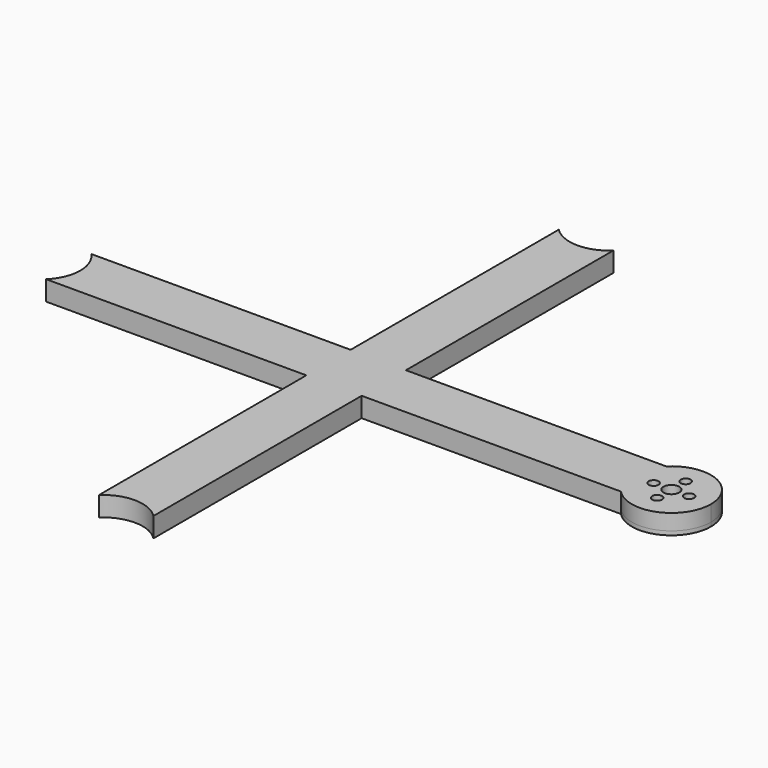
from build123d import *

# Parameters (mm, degrees)
F0_R     = 1.25
F0_R_2   = 2
F1_DEPTH = 5
F2_DEPTH = 1


with BuildPart() as f1:
    # F0 (on Top) → F1 (new body)
    with BuildSketch(Plane.XY):
        with BuildLine():
            ThreePointArc((72.7387571288, -6.8756346591), (83.7005115381, -9.2901137967), (90, 0))
            ThreePointArc((90, 0), (83.861757699, 9.2242521363), (72.9826345051, 7.1243653409))
            ThreePointArc((72.9826345051, 7.1243653409), (70.0015169041, 0.1741717018), (72.7387571288, -6.8756346591))
        make_face()
        with Locations((75.5, 0)):
            Circle(F0_R, mode=Mode.SUBTRACT)
        with Locations((80, -4.5)):
            Circle(F0_R, mode=Mode.SUBTRACT)
        with Locations((80, 0)):
            Circle(F0_R_2, mode=Mode.SUBTRACT)
        with Locations((84.5, 0)):
            Circle(F0_R, mode=Mode.SUBTRACT)
        with Locations((80, 4.5)):
            Circle(F0_R, mode=Mode.SUBTRACT)
        with BuildLine():
            ThreePointArc((72.7387571288, -6.8756346591), (70.0015169041, 0.1741717018), (72.9826345051, 7.1243653409))
            Line((72.9826345051, 7.1243653409), (7.1243653409, 7.1243653409))
            Line((7.1243653409, 7.1243653409), (7.1243653409, 0.2487306818))
            Line((7.1243653409, 0.2487306818), (7.1243653409, 0))
            Line((7.1243653409, 0), (7.1243653409, -6.8756346591))
            Line((7.1243653409, -6.8756346591), (72.7387571288, -6.8756346591))
        make_face()
        Polygon((7.1243653409, 0.2487306818), (7.1243653409, 7.1243653409), (0.2487306818, 7.1243653409), (0, 7.1243653409), (-6.8756346591, 7.1243653409), (-6.8756346591, 0.2487306818), (-6.8756346591, 0), (-6.8756346591, -6.8756346591), (0, -6.8756346591), (0.2487306818, -6.8756346591), (7.1243653409, -6.8756346591), (7.1243653409, 0), align=None)
        with BuildLine():
            Line((0.2487306818, 7.1243653409), (7.1243653409, 7.1243653409))
            Line((7.1243653409, 7.1243653409), (7.1243653409, 72.7387571288))
            ThreePointArc((7.1243653409, 72.7387571288), (0.0745589801, 70.0015169041), (-6.8756346591, 72.9826345051))
            Line((-6.8756346591, 72.9826345051), (-6.8756346591, 7.1243653409))
            Line((-6.8756346591, 7.1243653409), (0, 7.1243653409))
            Line((0, 7.1243653409), (0.2487306818, 7.1243653409))
        make_face()
        with BuildLine():
            Line((7.1243653409, -72.7339038233), (7.1243653409, -6.8756346591))
            Line((7.1243653409, -6.8756346591), (0.2487306818, -6.8756346591))
            Line((0.2487306818, -6.8756346591), (0, -6.8756346591))
            Line((0, -6.8756346591), (-6.8756346591, -6.8756346591))
            Line((-6.8756346591, -6.8756346591), (-6.8756346591, -72.4900264469))
            ThreePointArc((-6.8756346591, -72.4900264469), (0.1741717018, -69.7527862223), (7.1243653409, -72.7339038233))
        make_face()
        with BuildLine():
            Line((-6.8756346591, 0.2487306818), (-6.8756346591, 7.1243653409))
            Line((-6.8756346591, 7.1243653409), (-72.4900264469, 7.1243653409))
            ThreePointArc((-72.4900264469, 7.1243653409), (-70.4611555214, 3.94924222), (-69.7512693182, 0.2487306818))
            ThreePointArc((-69.7512693182, 0.2487306818), (-70.5270171818, -3.6130270171), (-72.7339038233, -6.8756346591))
            Line((-72.7339038233, -6.8756346591), (-6.8756346591, -6.8756346591))
            Line((-6.8756346591, -6.8756346591), (-6.8756346591, 0))
            Line((-6.8756346591, 0), (-6.8756346591, 0.2487306818))
        make_face()
    extrude(amount=F1_DEPTH)


with BuildPart() as f2:
    # F0 (on Top) → F2 (new body)
    with BuildSketch(Plane.XY):
        with BuildLine():
            ThreePointArc((72.7387571288, -6.8756346591), (83.7005115381, -9.2901137967), (90, 0))
            ThreePointArc((90, 0), (83.861757699, 9.2242521363), (72.9826345051, 7.1243653409))
            ThreePointArc((72.9826345051, 7.1243653409), (70.0015169041, 0.1741717018), (72.7387571288, -6.8756346591))
        make_face()
        with Locations((75.5, 0)):
            Circle(F0_R, mode=Mode.SUBTRACT)
        with Locations((80, -4.5)):
            Circle(F0_R, mode=Mode.SUBTRACT)
        with Locations((80, 0)):
            Circle(F0_R_2, mode=Mode.SUBTRACT)
        with Locations((84.5, 0)):
            Circle(F0_R, mode=Mode.SUBTRACT)
        with Locations((80, 4.5)):
            Circle(F0_R, mode=Mode.SUBTRACT)
    extrude(amount=F2_DEPTH)


solid = Compound([f1.part, f2.part])
